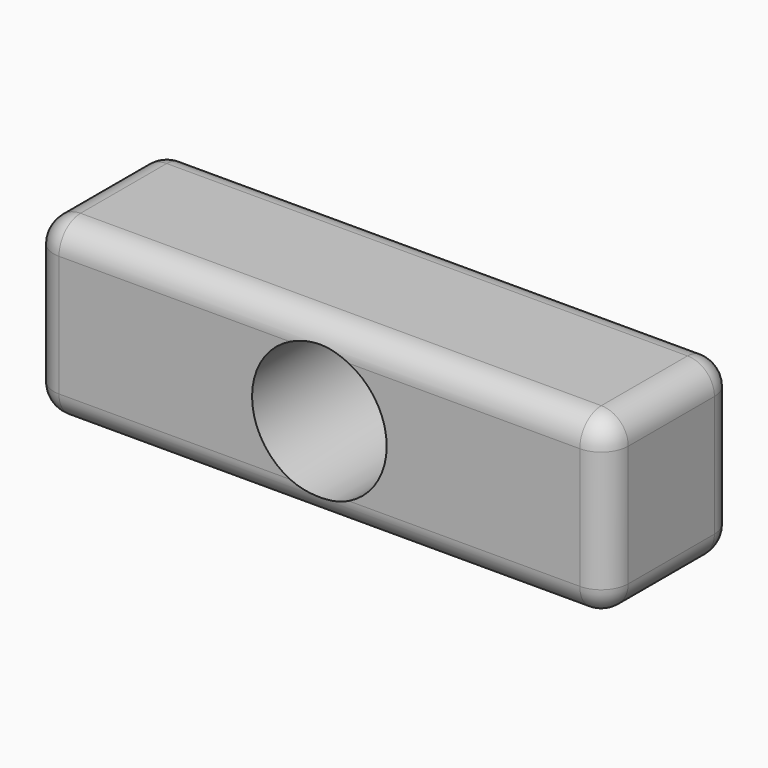
from build123d import *

# Parameters (mm, degrees)
F0_W         = 42.6834902611
F0_H         = 13
F0_R         = 5
F1_DEPTH     = 12
F2_T1_DEPTH  = 8
F2_T3_DEPTH  = 9
F2_T5_DEPTH  = 38.6834902611
F2_S9_W      = 2
F2_S9_H      = 2
F2_T10_DEPTH = 2
F2_S15_W     = 2
F2_S15_H     = 2
F2_T16_DEPTH = 2
F2_S21_W     = 2
F2_S21_H     = 2
F2_T22_DEPTH = 2
F2_S27_W     = 2
F2_S27_H     = 2
F2_T28_DEPTH = 2
F2_S33_W     = 2
F2_S33_H     = 2
F2_T34_DEPTH = 2
F2_S39_W     = 2
F2_S39_H     = 2
F2_T40_DEPTH = 2
F2_S45_W     = 2
F2_S45_H     = 2
F2_T46_DEPTH = 2
F2_S51_W     = 2
F2_S51_H     = 2
F2_T52_DEPTH = 2


# Not quite as in the source:
# - a fillet or chamfer that OpenCascade refuses, or shapes differently, is made with other operations: its cross-section is extruded or revolved along the edge and cut away or added


with BuildPart() as f1:
    # F0 (on Front) → F1 (new body)
    with BuildSketch(Plane.XZ):
        Rectangle(F0_W, F0_H)
        Circle(F0_R, mode=Mode.SUBTRACT)
    extrude(amount=F1_DEPTH)

    # F2: fillet of radius 2 on 13 edges, made by hand

    # F2_s2 → F2_t1 (cut)
    with BuildSketch(Plane.XZ.offset(2)):
        with BuildLine():
            ThreePointArc((-19.3417451306, 6.5), (-20.7559586929, 5.9142135624), (-21.3417451306, 4.5))
            Line((-21.3417451306, 4.5), (-21.3417451306, 6.5))
            Line((-21.3417451306, 6.5), (-19.3417451306, 6.5))
        make_face()
        with BuildLine():
            ThreePointArc((19.3417451306, 6.5), (20.7559586929, 5.9142135624), (21.3417451306, 4.5))
            Line((21.3417451306, 4.5), (21.3417451306, 6.5))
            Line((21.3417451306, 6.5), (19.3417451306, 6.5))
        make_face()
        with BuildLine():
            ThreePointArc((19.3417451306, -6.5), (20.7559586929, -5.9142135624), (21.3417451306, -4.5))
            Line((21.3417451306, -4.5), (21.3417451306, -6.5))
            Line((21.3417451306, -6.5), (19.3417451306, -6.5))
        make_face()
        with BuildLine():
            ThreePointArc((-21.3417451306, -4.5), (-20.7559586929, -5.9142135624), (-19.3417451306, -6.5))
            Line((-19.3417451306, -6.5), (-21.3417451306, -6.5))
            Line((-21.3417451306, -6.5), (-21.3417451306, -4.5))
        make_face()
    extrude(amount=F2_T1_DEPTH, mode=Mode.SUBTRACT)

    # F2_s4 → F2_t3 (cut)
    with BuildSketch(Plane.XY.offset(-4.5)):
        with BuildLine():
            ThreePointArc((21.3417451306, -10), (20.7559586929, -11.4142135624), (19.3417451306, -12))
            Line((19.3417451306, -12), (21.3417451306, -12))
            Line((21.3417451306, -12), (21.3417451306, -10))
        make_face()
        with BuildLine():
            ThreePointArc((21.3417451306, -2), (20.7559586929, -0.5857864376), (19.3417451306, 0))
            Line((19.3417451306, 0), (21.3417451306, 0))
            Line((21.3417451306, 0), (21.3417451306, -2))
        make_face()
        with BuildLine():
            ThreePointArc((-21.3417451306, -10), (-20.7559586929, -11.4142135624), (-19.3417451306, -12))
            Line((-19.3417451306, -12), (-21.3417451306, -12))
            Line((-21.3417451306, -12), (-21.3417451306, -10))
        make_face()
        with BuildLine():
            ThreePointArc((-21.3417451306, -2), (-20.7559586929, -0.5857864376), (-19.3417451306, 0))
            Line((-19.3417451306, 0), (-21.3417451306, 0))
            Line((-21.3417451306, 0), (-21.3417451306, -2))
        make_face()
    extrude(amount=F2_T3_DEPTH, mode=Mode.SUBTRACT)

    # F2_s6 → F2_t5 (cut)
    with BuildSketch(Plane.YZ.offset(-19.3417451306)):
        with BuildLine():
            ThreePointArc((-2, 6.5), (-0.5857864376, 5.9142135624), (0, 4.5))
            Line((0, 4.5), (0, 6.5))
            Line((0, 6.5), (-2, 6.5))
        make_face()
        with BuildLine():
            ThreePointArc((-10, 6.5), (-11.4142135624, 5.9142135624), (-12, 4.5))
            Line((-12, 4.5), (-12, 6.5))
            Line((-12, 6.5), (-10, 6.5))
        make_face()
        with BuildLine():
            ThreePointArc((-2, -6.5), (-0.5857864376, -5.9142135624), (0, -4.5))
            Line((0, -4.5), (0, -6.5))
            Line((0, -6.5), (-2, -6.5))
        make_face()
        with BuildLine():
            ThreePointArc((-10, -6.5), (-11.4142135624, -5.9142135624), (-12, -4.5))
            Line((-12, -4.5), (-12, -6.5))
            Line((-12, -6.5), (-10, -6.5))
        make_face()
    extrude(amount=F2_T5_DEPTH, mode=Mode.SUBTRACT)


with BuildPart() as f2_tool8:
    # F2_s9 → F2_t10 (new body)
    with BuildSketch(Plane.XY.offset(4.5)):
        with Locations((-20.3417451306, -1)):
            Rectangle(F2_S9_W, F2_S9_H)
    extrude(amount=F2_T10_DEPTH)

    # F2_s11 → F2_t12 (revolve, cut)
    with BuildSketch(Plane(origin=(-19.3417451306, -2, 4.5), x_dir=(0.7071067812, -0.7071067812, 0), z_dir=(-0.7071067812, -0.7071067812, 0))):
        with BuildLine():
            ThreePointArc((0, -2), (2, 0), (0, 2))
            Line((0, 2), (0, -2))
        make_face()
    revolve(axis=Axis((-19.3417451306, -2, 4.5), (0, 0, 1)), mode=Mode.SUBTRACT)


with BuildPart() as f1_1:
    add(f1.part)

    # F2_t7: cut F2_tool8
    add(f2_tool8.part, mode=Mode.SUBTRACT)


with BuildPart() as f2_tool14:
    # F2_s15 → F2_t16 (new body)
    with BuildSketch(Plane.XY.offset(4.5)):
        with Locations((-20.3417451306, -11)):
            Rectangle(F2_S15_W, F2_S15_H)
    extrude(amount=F2_T16_DEPTH)

    # F2_s17 → F2_t18 (revolve, cut)
    with BuildSketch(Plane(origin=(-19.3417451306, -10, 4.5), x_dir=(0.7071067812, 0.7071067812, 0), z_dir=(0.7071067812, -0.7071067812, 0))):
        with BuildLine():
            ThreePointArc((0, -2), (2, 0), (0, 2))
            Line((0, 2), (0, -2))
        make_face()
    revolve(axis=Axis((-19.3417451306, -10, 4.5), (0, 0, 1)), mode=Mode.SUBTRACT)


with BuildPart() as f1_2:
    add(f1_1.part)

    # F2_t13: cut F2_tool14
    add(f2_tool14.part, mode=Mode.SUBTRACT)


with BuildPart() as f2_tool20:
    # F2_s21 → F2_t22 (new body)
    with BuildSketch(Plane.XY.offset(4.5)):
        with Locations((20.3417451306, -1)):
            Rectangle(F2_S21_W, F2_S21_H)
    extrude(amount=F2_T22_DEPTH)

    # F2_s23 → F2_t24 (revolve, cut)
    with BuildSketch(Plane(origin=(19.3417451306, -2, 4.5), x_dir=(-0.7071067812, -0.7071067812, 0), z_dir=(-0.7071067812, 0.7071067812, 0))):
        with BuildLine():
            ThreePointArc((0, -2), (2, 0), (0, 2))
            Line((0, 2), (0, -2))
        make_face()
    revolve(axis=Axis((19.3417451306, -2, 4.5), (0, 0, 1)), mode=Mode.SUBTRACT)


with BuildPart() as f1_3:
    add(f1_2.part)

    # F2_t19: cut F2_tool20
    add(f2_tool20.part, mode=Mode.SUBTRACT)


with BuildPart() as f2_tool26:
    # F2_s27 → F2_t28 (new body)
    with BuildSketch(Plane.XY.offset(4.5)):
        with Locations((20.3417451306, -11)):
            Rectangle(F2_S27_W, F2_S27_H)
    extrude(amount=F2_T28_DEPTH)

    # F2_s29 → F2_t30 (revolve, cut)
    with BuildSketch(Plane(origin=(19.3417451306, -10, 4.5), x_dir=(-0.7071067812, 0.7071067812, 0), z_dir=(0.7071067812, 0.7071067812, 0))):
        with BuildLine():
            ThreePointArc((0, -2), (2, 0), (0, 2))
            Line((0, 2), (0, -2))
        make_face()
    revolve(axis=Axis((19.3417451306, -10, 4.5), (0, 0, 1)), mode=Mode.SUBTRACT)


with BuildPart() as f1_4:
    add(f1_3.part)

    # F2_t25: cut F2_tool26
    add(f2_tool26.part, mode=Mode.SUBTRACT)


with BuildPart() as f2_tool32:
    # F2_s33 → F2_t34 (new body)
    with BuildSketch(Plane.XY.offset(-4.5)):
        with Locations((20.3417451306, -1)):
            Rectangle(F2_S33_W, F2_S33_H)
    extrude(amount=-F2_T34_DEPTH)

    # F2_s35 → F2_t36 (revolve, cut)
    with BuildSketch(Plane(origin=(19.3417451306, -2, -4.5), x_dir=(-0.7071067812, -0.7071067812, 0), z_dir=(0.7071067812, -0.7071067812, 0))):
        with BuildLine():
            ThreePointArc((0, -2), (2, 0), (0, 2))
            Line((0, 2), (0, -2))
        make_face()
    revolve(axis=Axis((19.3417451306, -2, -4.5), (0, 0, -1)), mode=Mode.SUBTRACT)


with BuildPart() as f1_5:
    add(f1_4.part)

    # F2_t31: cut F2_tool32
    add(f2_tool32.part, mode=Mode.SUBTRACT)


with BuildPart() as f2_tool38:
    # F2_s39 → F2_t40 (new body)
    with BuildSketch(Plane.XY.offset(-4.5)):
        with Locations((20.3417451306, -11)):
            Rectangle(F2_S39_W, F2_S39_H)
    extrude(amount=-F2_T40_DEPTH)

    # F2_s41 → F2_t42 (revolve, cut)
    with BuildSketch(Plane(origin=(19.3417451306, -10, -4.5), x_dir=(-0.7071067812, 0.7071067812, 0), z_dir=(-0.7071067812, -0.7071067812, 0))):
        with BuildLine():
            ThreePointArc((0, -2), (2, 0), (0, 2))
            Line((0, 2), (0, -2))
        make_face()
    revolve(axis=Axis((19.3417451306, -10, -4.5), (0, 0, -1)), mode=Mode.SUBTRACT)


with BuildPart() as f1_6:
    add(f1_5.part)

    # F2_t37: cut F2_tool38
    add(f2_tool38.part, mode=Mode.SUBTRACT)


with BuildPart() as f2_tool44:
    # F2_s45 → F2_t46 (new body)
    with BuildSketch(Plane.YZ.offset(-19.3417451306)):
        with Locations((-11, -5.5)):
            Rectangle(F2_S45_W, F2_S45_H)
    extrude(amount=-F2_T46_DEPTH)

    # F2_s47 → F2_t48 (revolve, cut)
    with BuildSketch(Plane(origin=(-19.3417451306, -10, -4.5), x_dir=(0, 0.7071067812, 0.7071067812), z_dir=(0, -0.7071067812, 0.7071067812))):
        with BuildLine():
            ThreePointArc((0, -2), (2, 0), (0, 2))
            Line((0, 2), (0, -2))
        make_face()
    revolve(axis=Axis((-19.3417451306, -10, -4.5), (-1, 0, 0)), mode=Mode.SUBTRACT)


with BuildPart() as f1_7:
    add(f1_6.part)

    # F2_t43: cut F2_tool44
    add(f2_tool44.part, mode=Mode.SUBTRACT)


with BuildPart() as f2_tool50:
    # F2_s51 → F2_t52 (new body)
    with BuildSketch(Plane.YZ.offset(-19.3417451306)):
        with Locations((-1, -5.5)):
            Rectangle(F2_S51_W, F2_S51_H)
    extrude(amount=-F2_T52_DEPTH)

    # F2_s53 → F2_t54 (revolve, cut)
    with BuildSketch(Plane(origin=(-19.3417451306, -2, -4.5), x_dir=(0, -0.7071067812, 0.7071067812), z_dir=(0, -0.7071067812, -0.7071067812))):
        with BuildLine():
            ThreePointArc((0, -2), (2, 0), (0, 2))
            Line((0, 2), (0, -2))
        make_face()
    revolve(axis=Axis((-19.3417451306, -2, -4.5), (-1, 0, 0)), mode=Mode.SUBTRACT)


with BuildPart() as f1_8:
    add(f1_7.part)

    # F2_t49: cut F2_tool50
    add(f2_tool50.part, mode=Mode.SUBTRACT)

    # F2_s55 → F2_t56 (revolve, cut)
    with BuildSketch(Plane.XY):
        with BuildLine():
            ThreePointArc((5, -2), (5.5857864376, -0.5857864376), (7, 0))
            Line((7, 0), (5, 0))
            Line((5, 0), (5, -2))
        make_face()
    revolve(axis=Axis((0, 0, 0), (0, -1, 0)), mode=Mode.SUBTRACT)


solid = f1_8.part
